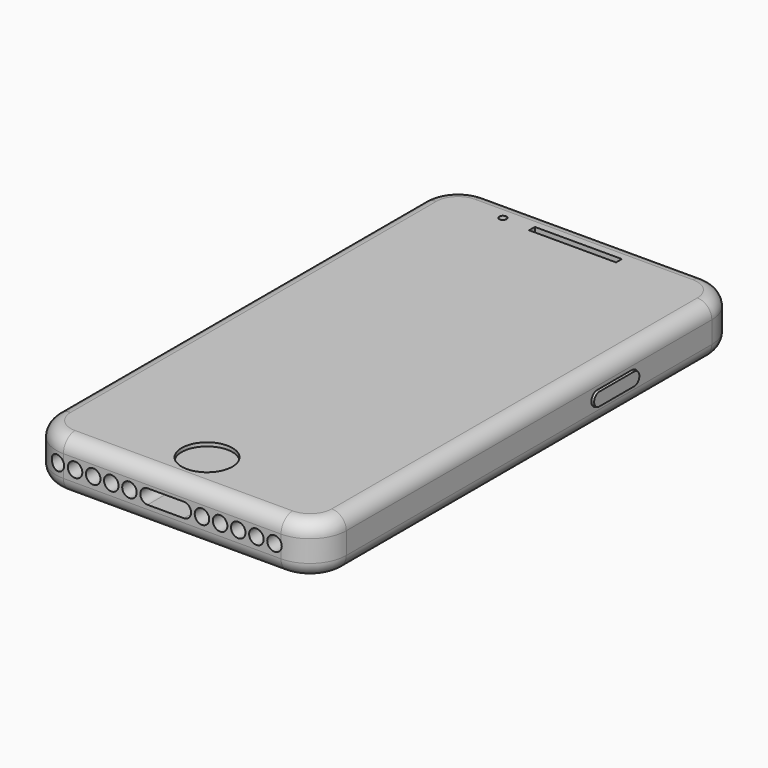
from build123d import *

# Parameters (mm, degrees)
F0_W         = 40
F0_H         = 73
F1_DEPTH     = 7
F3_R         = 1.0007571232
F4_DEPTH     = 8
F6_DEPTH     = 2
F8_DEPTH     = 2.3
F9_R         = 3.5
F10_DEPTH    = 0.5
F11_W        = 12
F11_H        = 1
F12_DEPTH    = 1
F13_T1_DEPTH = 32
F14_R        = 2
F15_R        = 2


# Not quite as in the source:
# - a fillet or chamfer that OpenCascade refuses, or shapes differently, is made with other operations: its cross-section is extruded or revolved along the edge and cut away or added


with BuildPart() as f1:
    # F0 (on Top) → F1 (new body)
    with BuildSketch(Plane.XY):
        with Locations((20, 36.5)):
            Rectangle(F0_W, F0_H)
    extrude(amount=F1_DEPTH)

    # F3 (on face) → F4 (cut)
    with BuildSketch(Plane.XZ):
        with Locations((4.10061609, 3.5689128563)):
            Circle(F3_R)
        with Locations((6.60061609, 3.5689128563)):
            Circle(F3_R)
        with Locations((9.10061609, 3.5689128563)):
            Circle(F3_R)
        with Locations((11.60061609, 3.5689128563)):
            Circle(F3_R)
        with Locations((14.10061609, 3.5689128563)):
            Circle(F3_R)
        with BuildLine():
            Line((21.60061609, 4.5696699795), (16.60061609, 4.5696699795))
            ThreePointArc((16.60061609, 4.5696699795), (15.5998589668, 3.5689128563), (16.60061609, 2.568155733))
            Line((16.60061609, 2.568155733), (21.60061609, 2.568155733))
            ThreePointArc((21.60061609, 2.568155733), (22.6013732132, 3.5689128563), (21.60061609, 4.5696699795))
        make_face()
        with Locations((24.10061609, 3.5689128563)):
            Circle(F3_R)
        with Locations((26.60061609, 3.5689128563)):
            Circle(F3_R)
        with Locations((29.10061609, 3.5689128563)):
            Circle(F3_R)
        with Locations((31.60061609, 3.5689128563)):
            Circle(F3_R)
        with Locations((34.10061609, 3.5689128563)):
            Circle(F3_R)
    extrude(amount=-F4_DEPTH, mode=Mode.SUBTRACT)

    # F5 (on face) → F6 (cut)
    with BuildSketch(Plane.YZ.offset(40)):
        with BuildLine():
            Line((54.2437834144, 4.5), (48.2437834144, 4.5))
            ThreePointArc((48.2437834144, 4.5), (47.2437834144, 3.5), (48.2437834144, 2.5))
            Line((48.2437834144, 2.5), (54.2437834144, 2.5))
            ThreePointArc((54.2437834144, 2.5), (55.2437834144, 3.5), (54.2437834144, 4.5))
        make_face()
    extrude(amount=-F6_DEPTH, mode=Mode.SUBTRACT)

    # F7 (on face) → F8 (join)
    with BuildSketch(Plane.YZ.offset(38)):
        with BuildLine():
            Line((54.2437834144, 4.4), (48.2437834144, 4.4))
            ThreePointArc((48.2437834144, 4.4), (47.3437834144, 3.5), (48.2437834144, 2.6))
            Line((48.2437834144, 2.6), (54.2437834144, 2.6))
            ThreePointArc((54.2437834144, 2.6), (55.1437834144, 3.5), (54.2437834144, 4.4))
        make_face()
    extrude(amount=F8_DEPTH)

    # F9 (on face) → F10 (cut)
    with BuildSketch(Plane.XY.offset(7)):
        with Locations((20, 6)):
            Circle(F9_R)
    extrude(amount=-F10_DEPTH, mode=Mode.SUBTRACT)

    # F11 (on face) → F12 (cut)
    with BuildSketch(Plane.XY.offset(7)):
        with Locations((20, 69.5)):
            Rectangle(F11_W, F11_H)
        with BuildLine():
            ThreePointArc((10.5, 69.5), (10.3535533906, 69.8535533906), (10, 70))
            Line((10, 70), (10, 69))
            ThreePointArc((10, 69), (10.3535533906, 69.1464466094), (10.5, 69.5))
        make_face()
        with BuildLine():
            Line((10, 69), (10, 70))
            ThreePointArc((10, 70), (9.5, 69.5), (10, 69))
        make_face()
    extrude(amount=-F12_DEPTH, mode=Mode.SUBTRACT)

    # F13: fillet of radius 5 on 4 edges, made by hand

    # F13_s2 → F13_t1 (cut)
    with BuildSketch(Plane.XY.offset(-12.5)):
        with BuildLine():
            ThreePointArc((35, 0), (38.5355339059, 1.4644660941), (40, 5))
            Line((40, 5), (40, 0))
            Line((40, 0), (35, 0))
        make_face()
        with BuildLine():
            ThreePointArc((0, 5), (1.4644660941, 1.4644660941), (5, 0))
            Line((5, 0), (0, 0))
            Line((0, 0), (0, 5))
        make_face()
        with BuildLine():
            ThreePointArc((35, 73), (38.5355339059, 71.5355339059), (40, 68))
            Line((40, 68), (40, 73))
            Line((40, 73), (35, 73))
        make_face()
        with BuildLine():
            ThreePointArc((0, 68), (1.4644660941, 71.5355339059), (5, 73))
            Line((5, 73), (0, 73))
            Line((0, 73), (0, 68))
        make_face()
    extrude(amount=F13_T1_DEPTH, mode=Mode.SUBTRACT)

    # F14
    f14_edges = [f1.edges().sort_by_distance(p)[0] for p in [
        (38.535534, 71.535534, 7),
        (20, 73, 7),
        (1.464466, 71.535534, 7),
        (0, 36.5, 7),
        (1.464466, 1.464466, 7),
        (20, 0, 7),
        (38.535534, 1.464466, 7),
        (40, 36.5, 7),
    ]]
    fillet(f14_edges, radius=F14_R)

    # F15
    f15_edges = [f1.edges().sort_by_distance(p)[0] for p in [
        (40, 36.5, 0),
        (38.535534, 71.535534, 0),
        (20, 73, 0),
        (1.464466, 71.535534, 0),
        (0, 36.5, 0),
        (38.535534, 1.464466, 0),
        (20, 0, 0),
        (1.464466, 1.464466, 0),
    ]]
    fillet(f15_edges, radius=F15_R)


solid = f1.part
